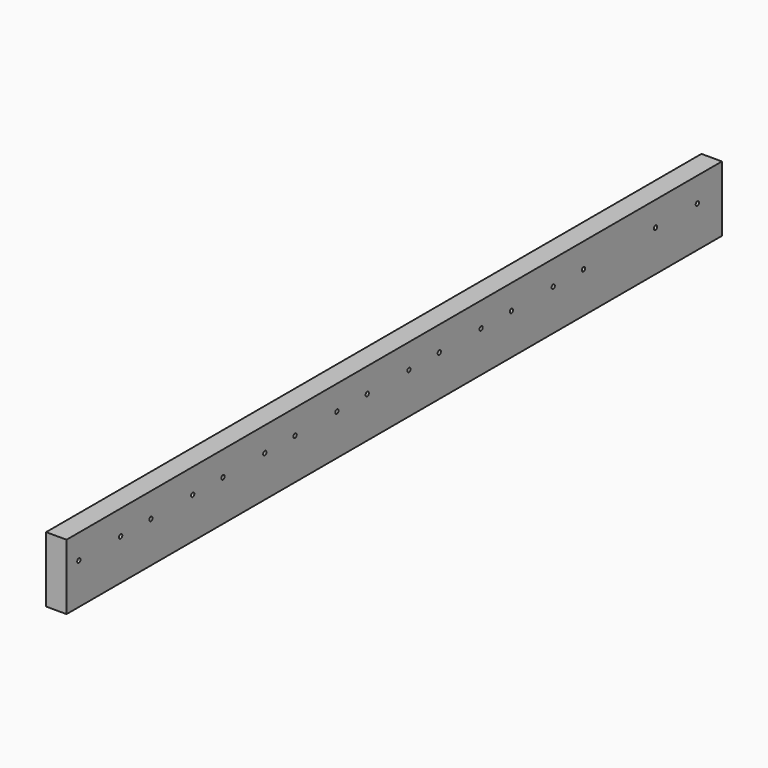
from build123d import *

# Parameters (mm, degrees)
F0_W     = 400
F0_H     = 32
F1_DEPTH = 10
F2_R     = 1
F3_DEPTH = 25


# Not quite as in the source:
# - a feature names something its author has since deleted; it is built from what else it names


with BuildPart() as f1:
    # F0 (on Right) → F1 (new body)
    with BuildSketch(Plane.YZ):
        Rectangle(F0_W, F0_H)
    extrude(amount=F1_DEPTH)

    # F2 (on face) → F3 (cut)
    with BuildSketch(Plane.YZ.offset(10)):
        with Locations((-192.5, 4)):
            Circle(F2_R)
        with Locations((-167, 4)):
            Circle(F2_R)
        with Locations((-148.5, 4)):
            Circle(F2_R)
        with Locations((-123, 4)):
            Circle(F2_R)
        with Locations((-104.5, 4)):
            Circle(F2_R)
        with Locations((-79, 4)):
            Circle(F2_R)
        with Locations((-60.5, 4)):
            Circle(F2_R)
        with Locations((-35, 4)):
            Circle(F2_R)
        with Locations((-16.5, 4)):
            Circle(F2_R)
        with Locations((9, 4)):
            Circle(F2_R)
        with Locations((27.5, 4)):
            Circle(F2_R)
        with Locations((53, 4)):
            Circle(F2_R)
        with Locations((71.5, 4)):
            Circle(F2_R)
        with Locations((97, 4)):
            Circle(F2_R)
        with Locations((115.5, 4)):
            Circle(F2_R)
        with Locations((159.5, 4)):
            Circle(F2_R)
        with Locations((185, 4)):
            Circle(F2_R)
    extrude(amount=-F3_DEPTH, mode=Mode.SUBTRACT)


solid = f1.part
